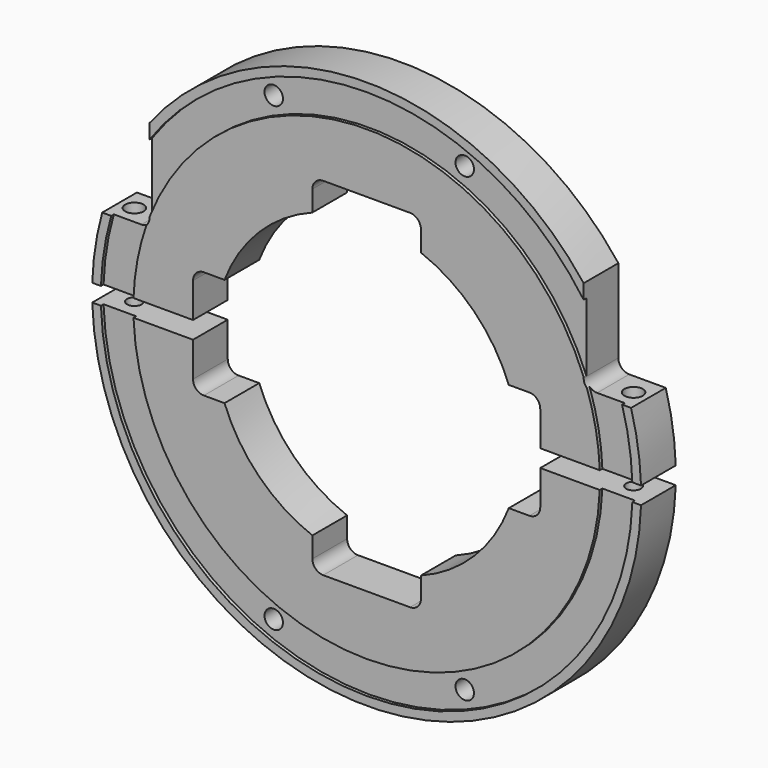
from build123d import *

# Parameters (mm, degrees)
F2_W     = 46.5
F2_H     = 8
F2_W_2   = 55
F2_H_2   = 21
F2_W_3   = 50
F2_H_3   = 55
F2_W_4   = 80
F2_H_4   = 80
F2_R     = 4.25
F3_DEPTH = 25
F5_D     = 6.8
F5_DEPTH = 22
F5_START = 4
F5_TIP   = 2.0429261047
F6_D     = 8.5
F6_DEPTH = 126.501
F7_R     = 5


with BuildPart() as f1:
    # F0 (on Right) → F1 (revolve)
    with BuildSketch(Plane.YZ):
        Polygon((20, 126.5), (0, 126.5), (0, 122.5), (1.5, 122.5), (1.5, 107.5), (0, 107.5), (0, 70.1), (20, 70.1), align=None)
    revolve(axis=Axis((0, 10, 0), (0, 1, 0)))

    # F2 (on Front) → F3 (cut)
    with BuildSketch(Plane.XZ):
        with Locations((-103.25, 0)):
            Rectangle(F2_W, F2_H)
        with Locations((-52.5, 14.5)):
            Rectangle(F2_W_2, F2_H_2)
        with Locations((-52.5, 0)):
            Rectangle(F2_W_2, F2_H)
        with Locations((0, 14.5)):
            Rectangle(F2_W_3, F2_H_2)
        with Locations((-52.5, -14.5)):
            Rectangle(F2_W_2, F2_H_2)
        with Locations((52.5, 14.5)):
            Rectangle(F2_W_2, F2_H_2)
        with Locations((52.5, 0)):
            Rectangle(F2_W_2, F2_H)
        with Locations((0, 52.5)):
            Rectangle(F2_W_3, F2_H_3)
        with Locations((0, -14.5)):
            Rectangle(F2_W_3, F2_H_2)
        with Locations((103.25, 0)):
            Rectangle(F2_W, F2_H)
        with Locations((52.5, -14.5)):
            Rectangle(F2_W_2, F2_H_2)
        with Locations((0, -52.5)):
            Rectangle(F2_W_3, F2_H_3)
        with Locations((-140, 74)):
            Rectangle(F2_W_4, F2_H_4)
        with Locations((140, 74)):
            Rectangle(F2_W_4, F2_H_4)
        with Locations((-44.008594722, 106.2461462388)):
            Circle(F2_R)
        with Locations((44.008594722, 106.2461462388)):
            Circle(F2_R)
        with Locations((-44.008594722, -106.2461462388)):
            Circle(F2_R)
        with Locations((44.008594722, -106.2461462388)):
            Circle(F2_R)
    extrude(amount=-F3_DEPTH, mode=Mode.SUBTRACT)

    # F5
    # its depths count from where the whole tool has entered the part; down to there all is cleared
    with Locations(Plane.XY.offset(-F5_START)):
        with Locations((-115, 10), (115, 10)):
            Hole(F5_D / 2, depth=F5_DEPTH)
            with Locations((0, 0, -(F5_DEPTH + F5_TIP / 2))):  # 118° drill point
                Cone(0, F5_D / 2, F5_TIP, mode=Mode.SUBTRACT)

    # F6 (through all, one way)
    with BuildSketch(Plane(origin=(0, 0, 0), x_dir=(1, 0, 0), z_dir=(0, 0, -1))):
        with Locations((-115, -10), (115, -10)):
            Circle(F6_D / 2)
    extrude(amount=-F6_DEPTH, mode=Mode.SUBTRACT)

    # F7
    f7_edges = [f1.edges().sort_by_distance(p)[0] for p in [
        (-80, 10, -25),
        (-80, 10, 25),
        (-25, 10, 80),
        (25, 10, 80),
        (80, 10, 25),
        (80, 10, -25),
        (25, 10, -80),
        (-25, 10, -80),
        (-100, 10, 34),
        (100, 10, 34),
    ]]
    fillet(f7_edges, radius=F7_R)


solid = f1.part
